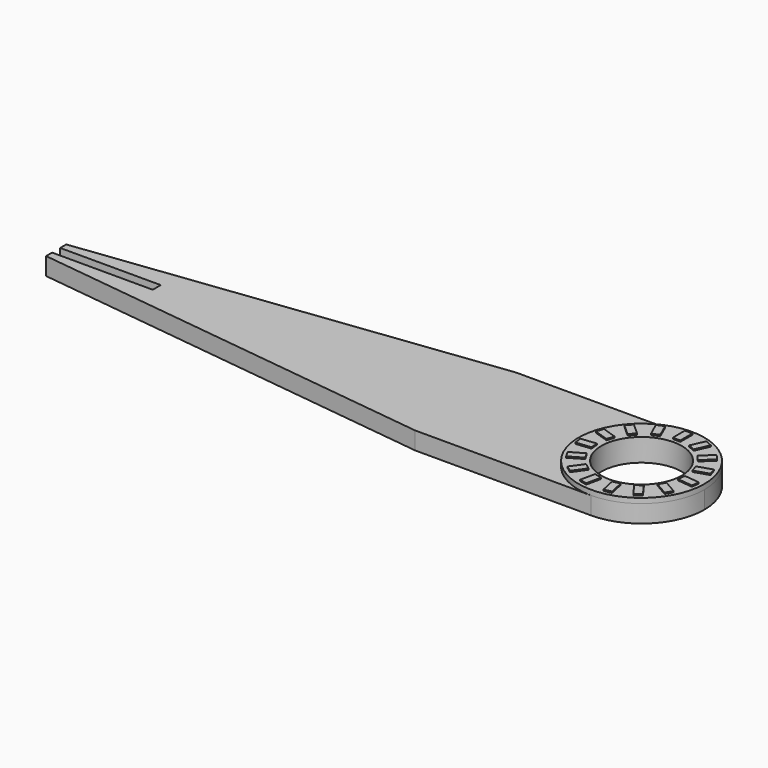
from build123d import *

# Parameters (mm, degrees)
F0_R         = 8
F1_DEPTH     = 3.5
F2_R         = 12.5
F2_R_2       = 8
F3_DEPTH     = 1
F4_W         = 20
F4_H         = 2
F5_DEPTH     = 1.75
F6_W         = 1.5
F6_H         = 3
F7_DEPTH     = 0.25
F8_TEXT_SIZE = 3.314394174
F9_DEPTH     = 0.25


# Not quite as in the source:
# - Text() gives the source's letters only with a copy of the font that has no kerning and outlines rounded to 1/6400 em; it was checked with that copy


with BuildPart() as f1:
    # F0 (on Top) → F1 (new body)
    with BuildSketch(Plane.XY):
        with BuildLine():
            ThreePointArc((0, -12.5), (8.8388347648, -8.8388347648), (12.5, 0))
            ThreePointArc((12.5, 0), (8.8388347648, 8.8388347648), (0, 12.5))
            ThreePointArc((0, 12.5), (-12.5, 0), (0, -12.5))
        make_face()
        Circle(F0_R, mode=Mode.SUBTRACT)
        with BuildLine():
            ThreePointArc((0, -12.5), (-12.5, 0), (0, 12.5))
            Line((0, 12.5), (-35, 12.5))
            Line((-35, 12.5), (-116.3887844346, 2.5067138408))
            Line((-116.3887844346, 2.5067138408), (-116.3887844346, -2.5067138408))
            Line((-116.3887844346, -2.5067138408), (-35, -12.5))
            Line((-35, -12.5), (0, -12.5))
        make_face()
    extrude(amount=F1_DEPTH)

    # F2 (on face) → F3 (join)
    with BuildSketch(Plane.XY.offset(3.5)):
        Circle(F2_R)
        Circle(F2_R_2, mode=Mode.SUBTRACT)
    extrude(amount=F3_DEPTH)

    # F4 (on face) → F5 (cut)
    with BuildSketch(Plane.XY.offset(3.5)):
        with Locations((-106.3887844346, -0.0067138408)):
            Rectangle(F4_W, F4_H)
    extrude(amount=-F5_DEPTH, mode=Mode.SUBTRACT)

    # F6 (on face) → F7 (join)
    with BuildSketch(Plane.XY.offset(4.5)):
        with Locations((-0.0151385421, 10.2250613223)):
            Rectangle(F6_W, F6_H)
        Polygon((-4.0976827353, 11.010271594), (-5.4680009217, 10.4001666294), (-4.2477909925, 7.6595302565), (-2.877472806, 8.2696352211), align=None)
        Polygon((-8.2217003572, 8.391705882), (-9.2253962667, 7.2769886438), (-6.9959617903, 5.2695968247), (-5.9922658807, 6.3843140629), align=None)
        Polygon((-10.9241112955, 4.3221379867), (-11.3876367871, 2.8955532123), (-8.5344672382, 1.9685022292), (-8.0709417466, 3.3950870036), align=None)
        Polygon((-11.7376441485, -0.4947668318), (-11.5808514535, -1.9865496749), (-8.5972857674, -1.6729642851), (-8.7540784623, -0.181181442), align=None)
        Polygon((-10.521631695, -5.2261219704), (-9.771631695, -6.5251600761), (-7.1735554836, -5.0251600761), (-7.9235554836, -3.7261219704), align=None)
        Polygon((-7.4863335354, -9.0538331424), (-6.2728080438, -9.9355110209), (-4.5094522869, -7.5084600377), (-5.7229777785, -6.6267821593), align=None)
        Polygon((-3.1565802963, -11.3160543126), (-1.6893588952, -11.6279218489), (-1.0656238228, -8.6934790467), (-2.5328452239, -8.3816115104), align=None)
        Polygon((1.7189743526, -11.6216268891), (3.1861957537, -11.3097593528), (2.5624606812, -8.3753165506), (1.0952392801, -8.6871840869), align=None)
        Polygon((6.2973027195, -9.9177145972), (7.5108282111, -9.0360367188), (5.7474724542, -6.6089857357), (4.5339469627, -7.4906636141), align=None)
        Polygon((9.7867702371, -6.4989393519), (10.5367702371, -5.1999012462), (7.9386940257, -3.6999012462), (7.1886940257, -4.9989393519), align=None)
        Polygon((11.5840162706, -1.9564384516), (11.7408089655, -0.4646556086), (8.7572432794, -0.1510702188), (8.6004505845, -1.6428530618), align=None)
        Polygon((11.3782806535, 2.9243484306), (10.9147551619, 4.3509332051), (8.0615856131, 3.4238822219), (8.5251111046, 1.9972974475), align=None)
        Polygon((9.2051369429, 7.2994889023), (8.2014410334, 8.4142061405), (5.972006557, 6.4068143215), (6.9757024665, 5.2920970833), align=None)
        Polygon((5.4403414289, 10.4124814291), (4.0700232424, 11.0225863937), (2.8498133132, 8.2819500207), (4.2201314997, 7.6718450561), align=None)
    extrude(amount=F7_DEPTH)

    # F8 (on face) → F9 (cut)
    with BuildSketch(Plane(origin=(0, 0, 0), x_dir=(1, 0, 0), z_dir=(0, 0, -1))):
        with Locations((-52.2852987051, -1.2500000885)):
            Text("Mr. Andrews's Compass", F8_TEXT_SIZE, font='Open Sans', text_align=(TextAlign.LEFT, TextAlign.BOTTOM))
    extrude(amount=-F9_DEPTH, mode=Mode.SUBTRACT)


solid = f1.part
